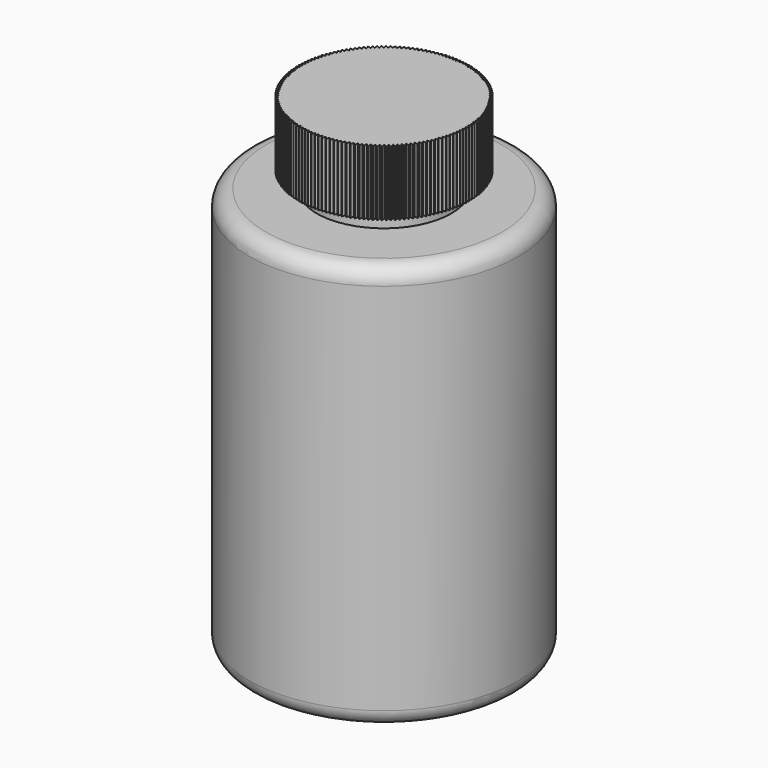
from build123d import *

# Parameters (mm, degrees)
F0_R             = 26.5565565878
F1_DEPTH         = 20.32
F2_R             = 21.086262788
F3_DEPTH         = 5.08
F5_R             = 42.0166917627
F6_DEPTH         = 127
F7_R             = 5.08
F9_DEPTH         = 25.4
F9_FACE_W        = 16.0293121402
F9_FACE_H        = 25.4
F16_DEPTH        = 20.32
F16_COPIES_COUNT = 150


# Not quite as in the source:
# - a pattern or mirror of a feature is missing from the dataset's text; its kind, count and spacing are read off the source's solid
# - a feature names something its author has since deleted; it is built from what else it names


with BuildPart() as f1:
    # F0 (on Top) → F1 (new body)
    with BuildSketch(Plane.XY):
        Circle(F0_R)
    extrude(amount=F1_DEPTH)

    # F2 (on Top) → F3 (join)
    with BuildSketch(Plane.XY):
        Circle(F2_R)
    extrude(amount=-F3_DEPTH)

    # F5 (on offset) → F6 (join)
    with BuildSketch(Plane.XY.offset(-5.08)):
        Circle(F5_R)
    extrude(amount=-F6_DEPTH)

    # F7
    f7_edges = [f1.edges().sort_by_distance(p)[0] for p in [
        (42.016692, 0, -68.58),
        (-42.016692, 0, -5.08),
        (-42.016692, 0, -132.08),
    ]]
    fillet(f7_edges, radius=F7_R)

    # F13 (on offset) → F16 (cut)
    with BuildSketch(Plane.XY.offset(20.32)):
        with BuildLine():
            ThreePointArc((-24.6199043172, -9.9554512308), (-24.4632311669, -10.4112297735), (-24.2433974956, -10.8401280282))
            Line((-24.2433974956, -10.8401280282), (-23.5797204077, -10.1301083341))
            Line((-23.5797204077, -10.1301083341), (-24.6199043172, -9.9554512308))
        make_face()
    f16 = extrude(amount=-F16_DEPTH, mode=Mode.SUBTRACT)

    # F16_copies: F16 ×150 about axis
    f16_copies_axis = Axis((0, 0, 0), (0, 0, 1))
    for i in range(1, F16_COPIES_COUNT):
        add(f16.rotate(f16_copies_axis, i * 360 / F16_COPIES_COUNT), mode=Mode.SUBTRACT)


with BuildPart() as f9:
    # F8 (on Top) → F9 (new body)
    with BuildSketch(Plane.XY):
        Polygon((-61.3985564099, 30.5373773032), (-54.405393125, 44.9607789464), (-65.9618569455, 56.0687486824), (-80.0973076611, 48.510449882), (-77.2770328292, 32.7311945903), align=None)
    extrude(amount=F9_DEPTH)

    # F11: sweep along a path in F10
    with BuildLine(Plane.XY) as f11_path:
        Line((-42.8944863379, 41.9798344374), (-26.6806501895, 62.3400732875))
    # F9_face (on face) → F11 (sweep)
    with BuildSketch(Plane(origin=(-73.0295823033, 52.2895992822, 12.7), x_dir=(-0.8818501126, -0.4715298282, 0), z_dir=(-0.4715298282, 0.8818501126, 0))):
        Rectangle(F9_FACE_W, F9_FACE_H)
    sweep(path=f11_path.line)


solid = f1.part
